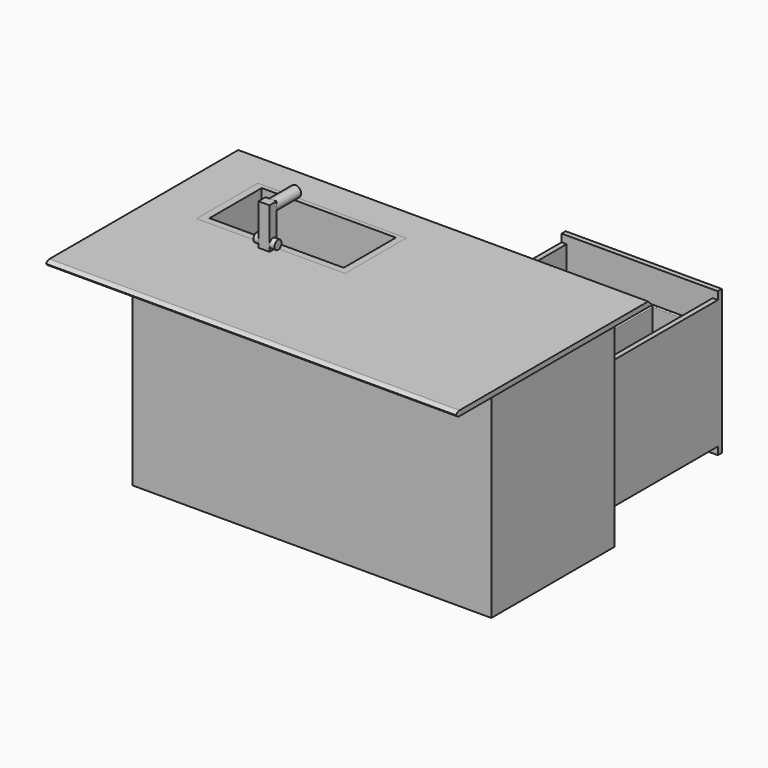
from build123d import *

# Parameters (mm, degrees)
F0_W         = 2032
F0_H         = 1270
F1_DEPTH     = 25.4
F2_W         = 1778
F2_H         = 762
F3_DEPTH     = 1066.8
F4_W         = 774.7
F4_H         = 122.7232557205
F5_DEPTH     = 25.4
F6_W         = 723.9
F6_H         = 71.9232557205
F7_DEPTH     = 5.08
F8_W         = 774.7
F8_H         = 715.4767442795
F9_DEPTH     = 25.4
F10_DEPTH    = 762
F11_W        = 736.6
F11_H        = 38.1
F12_DEPTH    = 787.4
F13_T        = -25.4
F14_W        = 723.9
F14_H        = 664.6767442795
F15_DEPTH    = 5.08
F16_W        = 723.9
F16_H        = 664.6767442795
F17_DEPTH    = 5.08
F18_T1_DEPTH = 2159
F19_T1_DEPTH = 2423.924487366
F20_W        = 508
F20_H        = 25.4
F21_DEPTH    = 127
F23_W        = 254
F23_H        = 584.2
F24_DEPTH    = 508
F25_T        = -12.7
F26_R        = 5.08
F27_W        = 735.7604503632
F27_H        = 380.0623416901
F28_DEPTH    = 254
F29_W        = 665.324151516
F29_H        = 323.6712217331
F30_DEPTH    = 228.6
F31_W        = 54.479598999
F31_H        = 43.5836911201
F32_DEPTH    = 203.2
F33_R        = 27.2397994995
F34_DEPTH    = 152.4
F35_R        = 22.0206677914
F36_DEPTH    = 25.4
F37_R        = 22.0203995705
F38_DEPTH    = 25.4


# Not quite as in the source:
# - a fillet or chamfer that OpenCascade refuses, or shapes differently, is made with other operations: its cross-section is extruded or revolved along the edge and cut away or added
# - a shell that OpenCascade refuses in one call is made with other operations: the cavity is built on its own and cut out


with BuildPart() as f1:
    # F0 (on Top) → F1 (new body)
    with BuildSketch(Plane.XY):
        with Locations((180.7471609741, 358.5185925256)):
            Rectangle(F0_W, F0_H)
    extrude(amount=F1_DEPTH)

    # F2 (on face) → F3 (join)
    with BuildSketch(Plane(origin=(0, 0, 0), x_dir=(1, 0, 0), z_dir=(0, 0, -1))):
        with Locations((180.7471609741, -485.5185925256)):
            Rectangle(F2_W, F2_H)
    extrude(amount=F3_DEPTH)

    # F4 (on face) → F5 (join)
    with BuildSketch(Plane(origin=(0, 866.5185925256, 0), x_dir=(-1, 0, 0), z_dir=(0, 1, 0))):
        with Locations((-606.1971609741, -137.5616278603)):
            Rectangle(F4_W, F4_H)
        with Locations((244.7028390259, -137.5616278603)):
            Rectangle(F4_W, F4_H)
    extrude(amount=F5_DEPTH)

    # F6 (on face) → F7 (cut)
    with BuildSketch(Plane(origin=(0, 891.9185925256, 0), x_dir=(-1, 0, 0), z_dir=(0, 1, 0))):
        with Locations((-606.1971609741, -137.5616278603)):
            Rectangle(F6_W, F6_H)
        with Locations((244.7028390259, -137.5616278603)):
            Rectangle(F6_W, F6_H)
    extrude(amount=-F7_DEPTH, mode=Mode.SUBTRACT)

    # F8 (on face) → F9 (join)
    with BuildSketch(Plane(origin=(0, 866.5185925256, 0), x_dir=(-1, 0, 0), z_dir=(0, 1, 0))):
        with Locations((244.7028390259, -632.8616278603)):
            Rectangle(F8_W, F8_H)
    extrude(amount=F9_DEPTH)

    # F8 (on face) → F10 (join)
    with BuildSketch(Plane(origin=(0, 866.5185925256, 0), x_dir=(-1, 0, 0), z_dir=(0, 1, 0))):
        with Locations((-606.1971609741, -632.8616278603)):
            Rectangle(F8_W, F8_H)
    extrude(amount=F10_DEPTH)

    # F11 (on face) → F12 (cut)
    with BuildSketch(Plane(origin=(218.8471609741, 0, 0), x_dir=(0, -1, 0), z_dir=(-1, 0, 0))):
        with Locations((-1234.8185925256, -294.1732557205)):
            Rectangle(F11_W, F11_H)
        with Locations((-1234.8185925256, -971.55)):
            Rectangle(F11_W, F11_H)
    extrude(amount=-F12_DEPTH, mode=Mode.SUBTRACT)

    # F13: a shell. OpenCascade refuses it in one call, so the cavity is built on its own and cut out:
    # the body offset inwards by the wall thickness, plus a prism from it out through each open face.
    f13_core = offset(f1.part, amount=F13_T, kind=Kind.INTERSECTION, mode=Mode.PRIVATE)
    f13_exits = [f13_core.faces().sort_by_distance(p)[0] for p in [
        (606.197161, 1222.118593, -338.623256),
    ]]
    add(f13_core, mode=Mode.SUBTRACT)
    extrude(f13_exits, amount=-F13_T, mode=Mode.SUBTRACT)

    # F14 (on face) → F15 (cut)
    with BuildSketch(Plane(origin=(0, 891.9185925256, 0), x_dir=(-1, 0, 0), z_dir=(0, 1, 0))):
        with Locations((244.7028390259, -632.8616278603)):
            Rectangle(F14_W, F14_H)
    extrude(amount=-F15_DEPTH, mode=Mode.SUBTRACT)

    # F16 (on face) → F17 (cut)
    with BuildSketch(Plane(origin=(0, 1628.5185925256, 0), x_dir=(-1, 0, 0), z_dir=(0, 1, 0))):
        with Locations((-606.1971609741, -632.8616278603)):
            Rectangle(F16_W, F16_H)
    extrude(amount=-F17_DEPTH, mode=Mode.SUBTRACT)

    # F18: fillet of radius 25.4 on 2 edges, made by hand

    # F18_s2 → F18_t1 (cut)
    with BuildSketch(Plane.YZ.offset(-898.7528390259)):
        with BuildLine():
            ThreePointArc((-251.0814074744, 25.4), (-269.0419197166, 17.9605122421), (-276.4814074744, 0))
            Line((-276.4814074744, 0), (-276.4814074744, 25.4))
            Line((-276.4814074744, 25.4), (-251.0814074744, 25.4))
        make_face()
        with BuildLine():
            ThreePointArc((-251.0814074744, 0), (-269.0419197166, 7.4394877579), (-276.4814074744, 25.4))
            Line((-276.4814074744, 25.4), (-276.4814074744, 0))
            Line((-276.4814074744, 0), (-251.0814074744, 0))
        make_face()
    extrude(amount=F18_T1_DEPTH, mode=Mode.SUBTRACT)

    # F19: chamfer of 76.2 on 1 edges, made by hand

    # F19_s2 → F19_t1 (cut)
    with BuildSketch(Plane.YZ.offset(-1031.2150827089)):
        Polygon((993.5185925256, -50.8), (917.3185925256, 25.4), (993.5185925256, 25.4), align=None)
    extrude(amount=F19_T1_DEPTH, mode=Mode.SUBTRACT)

    # F20 (on face) → F21 (join)
    with BuildSketch(Plane.YZ.offset(244.2471609741)):
        with Locations((1222.1185925256, -452.9232557205)):
            Rectangle(F20_W, F20_H)
    extrude(amount=F21_DEPTH)


with BuildPart() as f24:
    # F23 (on offset) → F24 (new body)
    with BuildSketch(Plane.XY.offset(-927.1)):
        with Locations((815.7471609741, 1285.6185925256)):
            Rectangle(F23_W, F23_H)
    extrude(amount=F24_DEPTH)

    # F25
    f25_openings = [f24.faces().sort_by_distance(p)[0] for p in [
        (815.747161, 1285.618593, -419.1),
    ]]
    offset(amount=F25_T, openings=f25_openings)

    # F26
    f26_edges = [f24.edges().sort_by_distance(p)[0] for p in [
        (688.747161, 1577.718593, -673.1),
        (942.747161, 1577.718593, -673.1),
        (688.747161, 993.518593, -673.1),
        (942.747161, 993.518593, -673.1),
        (942.747161, 1285.618593, -419.1),
        (930.047161, 1285.618593, -419.1),
        (815.747161, 1577.718593, -419.1),
        (815.747161, 1565.018593, -419.1),
        (701.447161, 1285.618593, -419.1),
        (688.747161, 1285.618593, -419.1),
        (815.747161, 1006.218593, -419.1),
        (815.747161, 993.518593, -419.1),
    ]]
    fillet(f26_edges, radius=F26_R)


with BuildPart() as f28:
    # F27 (on face) → F28 (new body)
    with BuildSketch(Plane.XY.offset(25.4)):
        with Locations((-233.930170536, 557.5037002563)):
            Rectangle(F27_W, F27_H)
    extrude(amount=-F28_DEPTH)


with BuildPart() as f30_tool:
    # F29 (on face) → F30 (new body)
    with BuildSketch(Plane.XY.offset(25.4)):
        with Locations((-232.4104309082, 563.6555552483)):
            Rectangle(F29_W, F29_H)
    extrude(amount=-F30_DEPTH)


with BuildPart() as f1_1:
    add(f1.part)

    # F30: cut by f30_tool
    add(f30_tool.part, mode=Mode.SUBTRACT)


with BuildPart() as f28_1:
    add(f28.part)

    # F30: cut by f30_tool
    add(f30_tool.part, mode=Mode.SUBTRACT)


with BuildPart() as f32:
    # F31 (on face) → F32 (new body)
    with BuildSketch(Plane.XY.offset(25.4)):
        with Locations((-234.6597015858, 348.1185734272)):
            Rectangle(F31_W, F31_H)
    extrude(amount=F32_DEPTH)

    # F33 (on face) → F34 (join)
    with BuildSketch(Plane(origin=(0, 369.9104189873, 0), x_dir=(-1, 0, 0), z_dir=(0, 1, 0))):
        with Locations((234.6597015858, 200.67730546)):
            Circle(F33_R)
    extrude(amount=F34_DEPTH)


with BuildPart() as f36:
    # F35 (on face) → F36 (new body)
    with BuildSketch(Plane(origin=(-261.8995010853, 0, 0), x_dir=(0, -1, 0), z_dir=(-1, 0, 0))):
        with Locations((-348.3473956585, 54.0832839906)):
            Circle(F35_R)
    extrude(amount=F36_DEPTH)


with BuildPart() as f38:
    # F37 (on face) → F38 (new body)
    with BuildSketch(Plane.YZ.offset(-207.4199020863)):
        with Locations((347.8900194168, 55.4691664875)):
            Circle(F37_R)
    extrude(amount=F38_DEPTH)


solid = Compound([f24.part, f1_1.part, f28_1.part, f32.part, f36.part, f38.part])
